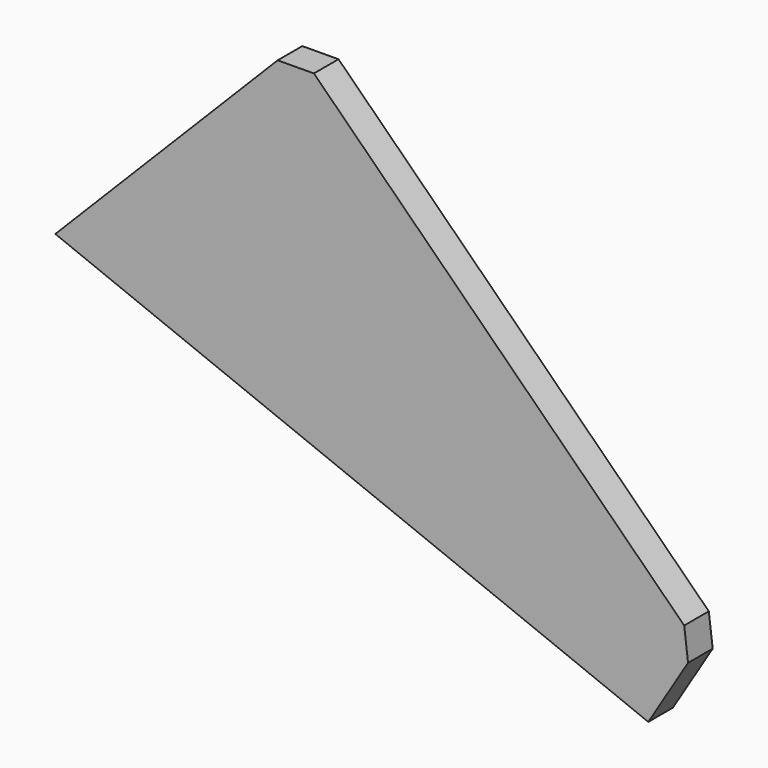
from build123d import *

# Parameters (mm, degrees)
F1_DEPTH    = 6
F2_T1_DEPTH = 31.7168298797
F2_T3_DEPTH = 26.6288680093


# Not quite as in the source:
# - a fillet or chamfer that OpenCascade refuses, or shapes differently, is made with other operations: its cross-section is extruded or revolved along the edge and cut away or added


with BuildPart() as f1:
    # F0 (on Front) → F1 (new body)
    with BuildSketch(Plane.XZ):
        Polygon((202.5005221367, 0), (155.6514501572, -47.4510490894), (271.2386846542, -93.6057344079), (281.0647502264, -77.5675406007), align=None)
    extrude(amount=F1_DEPTH)

    # F2: chamfer of 5 on 2 edges, made by hand

    # F2_s2 → F2_t1 (cut)
    with BuildSketch(Plane.XZ.offset(-12.8584149398)):
        Polygon((198.9876293479, -3.5580309518), (206.0585530885, -3.5128927888), (202.5005221367, 0), align=None)
    extrude(amount=F2_T1_DEPTH, mode=Mode.SUBTRACT)

    # F2_s4 → F2_t3 (cut)
    with BuildSketch(Plane.XZ.offset(-10.3144340046)):
        Polygon((278.9922098799, -80.9503598488), (278.2416469809, -74.7802520225), (281.0647502264, -77.5675406007), align=None)
    extrude(amount=F2_T3_DEPTH, mode=Mode.SUBTRACT)


solid = f1.part
